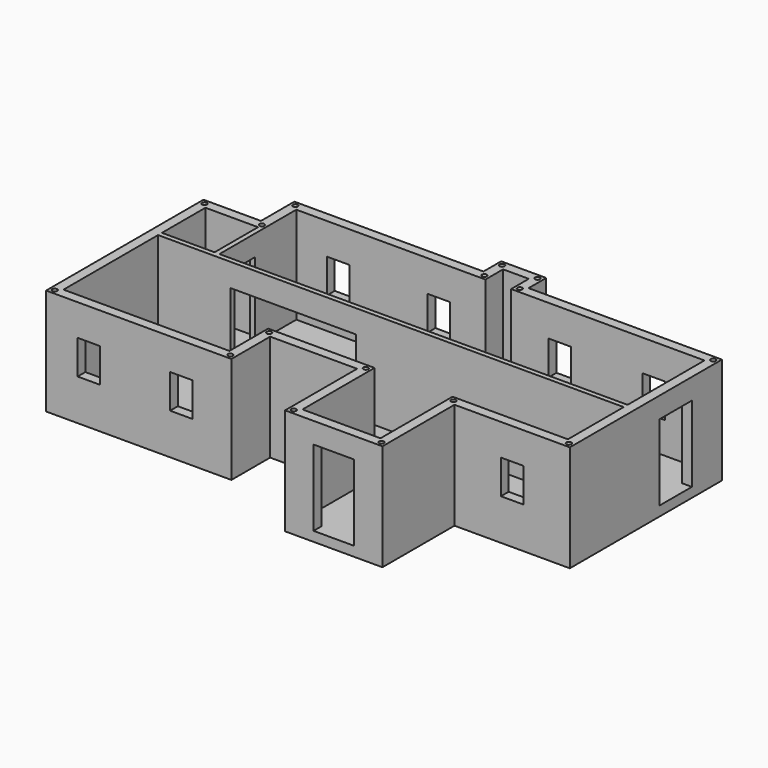
from build123d import *

# Parameters (mm, degrees)
F0_R      = 0.6477
F0_R_2    = 0.6441405576
F0_W      = 1.27
F0_H      = 14.2598937347
F2_DEPTH  = 25.4
F12_DEPTH = 2.54
F4_W      = 5.8928
F4_H      = 8.9408
F3_W      = 5.8928
F3_H      = 8.9408
F13_DEPTH = 25.4
F6_W      = 5.8928
F6_H      = 8.9408
F5_W      = 10.5937230855
F5_H      = 19.9419036508
F7_W      = 5.8928
F7_H      = 8.9408
F14_DEPTH = 12.7
F10_W     = 10.5918
F10_H     = 19.939
F15_DEPTH = 12.7
F9_W      = 10.5918
F9_H      = 19.939
F16_DEPTH = 25.4
F8_W      = 32.9645648599
F8_H      = 19.3392261863
F17_DEPTH = 12.7


# Not quite as in the source:
# - the program builds the solid bodies; features that only make, move or delete a surface that nothing else refers to are left out


with BuildPart() as f2:
    # F0 (on Top) → F2 (new body)
    with BuildSketch(Plane.XY):
        Polygon((-45.4049956864, 2.54), (-47.9449956864, 2.54), (-47.9449956864, 0), (-47.9449956864, -8.4182334522), (-60.4807920754, -8.4182334522), (-63.0207920754, -8.4182334522), (-63.0207920754, -10.9582334522), (-63.0207920754, -57.4975824572), (-63.0207920754, -60.0375824572), (-60.4807920754, -60.0375824572), (-16.9454139954, -60.0375824572), (-14.4054139954, -60.0375824572), (-14.4054139954, -57.4975824572), (-14.4054139954, -47.3375824572), (8.416604454, -47.3375824572), (8.416604454, -68.4223124651), (8.416604454, -70.9623124651), (10.956604454, -70.9623124651), (31.4210504293, -70.9623124651), (33.9610504293, -70.9623124651), (33.9610504293, -68.4223124651), (33.9610504293, -47.3375824572), (61.6818144917, -47.3375824572), (64.2218144917, -47.3375824572), (64.2218144917, -44.7975824572), (64.2218144917, 0), (64.2218144917, 2.54), (61.6818144917, 2.54), (13.496604454, 2.54), (13.496604454, 5.7937128431), (13.496604454, 8.3337128431), (10.956604454, 8.3337128431), (4.2076310147, 8.3337128431), (1.6676310147, 8.3337128431), (1.6676310147, 5.7937128431), (1.6676310147, 2.54), align=None)
        with Locations((-61.7507920754, -58.7675824572)):
            Circle(F0_R, mode=Mode.SUBTRACT)
        with Locations((-15.6754139954, -58.7675824572)):
            Circle(F0_R, mode=Mode.SUBTRACT)
        with Locations((-15.6754139954, -46.0675824572)):
            Circle(F0_R, mode=Mode.SUBTRACT)
        with Locations((9.686604454, -69.6923124651)):
            Circle(F0_R, mode=Mode.SUBTRACT)
        with Locations((32.6910504293, -69.6923124651)):
            Circle(F0_R, mode=Mode.SUBTRACT)
        with Locations((9.686604454, -46.0675824572)):
            Circle(F0_R, mode=Mode.SUBTRACT)
        with Locations((32.6910504293, -46.0675824572)):
            Circle(F0_R, mode=Mode.SUBTRACT)
        with Locations((62.9518144917, -46.0675824572)):
            Circle(F0_R, mode=Mode.SUBTRACT)
        with Locations((-61.7507920754, -9.6882334522)):
            Circle(F0_R, mode=Mode.SUBTRACT)
        with Locations((-46.6749956864, -9.6882334522)):
            Circle(F0_R, mode=Mode.SUBTRACT)
        with Locations((-46.6749956864, 1.27)):
            Circle(F0_R_2, mode=Mode.SUBTRACT)
        Polygon((10.956604454, -68.4223124651), (10.956604454, -47.3375824572), (10.956604454, -44.7975824572), (8.416604454, -44.7975824572), (-14.4054139954, -44.7975824572), (-16.9454139954, -44.7975824572), (-16.9454139954, -47.3375824572), (-16.9454139954, -57.4975824572), (-60.4807920754, -57.4975824572), (-60.4807920754, -26.4881271869), (-60.4807920754, -25.2181271869), (-60.4807920754, -10.9582334522), (-47.9449956864, -10.9582334522), (-46.6749956864, -10.9582334522), (-45.4049956864, -10.9582334522), (-45.4049956864, -8.4182334522), (-45.4049956864, 0), (1.6676310147, 0), (4.2076310147, 0), (4.2076310147, 2.54), (4.2076310147, 5.7937128431), (10.956604454, 5.7937128431), (10.956604454, 2.54), (10.956604454, 0), (13.496604454, 0), (61.6818144917, 0), (61.6818144917, -25.2181271869), (61.6818144917, -26.4881271869), (61.6818144917, -44.7975824572), (33.9610504293, -44.7975824572), (31.4210504293, -44.7975824572), (31.4210504293, -47.3375824572), (31.4210504293, -68.4223124651), align=None, mode=Mode.SUBTRACT)
        with Locations((2.9376310147, 1.27)):
            Circle(F0_R, mode=Mode.SUBTRACT)
        with Locations((12.226604454, 1.27)):
            Circle(F0_R, mode=Mode.SUBTRACT)
        with Locations((2.9376310147, 7.0637128431)):
            Circle(F0_R, mode=Mode.SUBTRACT)
        with Locations((12.226604454, 7.0637128431)):
            Circle(F0_R, mode=Mode.SUBTRACT)
        with Locations((62.9518144917, 1.27)):
            Circle(F0_R, mode=Mode.SUBTRACT)
        Polygon((-60.4807920754, -26.4881271869), (61.6818144917, -26.4881271869), (61.6818144917, -25.2181271869), (-45.4049956864, -25.2181271869), (-46.6749956864, -25.2181271869), (-60.4807920754, -25.2181271869), align=None)
        with Locations((-46.0399956864, -18.0881803195)):
            Rectangle(F0_W, F0_H)
    extrude(amount=F2_DEPTH)

    # F11 (on face) → F12 (join)
    with BuildSketch(Plane(origin=(0, 0, 0), x_dir=(1, 0, 0), z_dir=(0, 0, -1))):
        Polygon((13.496604454, -8.3337128431), (13.496604454, -2.54), (64.2218144917, -2.54), (64.2218144917, 47.3375824572), (33.9610504293, 47.3375824572), (33.9610504293, 70.9623124651), (8.416604454, 70.9623124651), (8.416604454, 47.3375824572), (-14.4054139954, 47.3375824572), (-14.4054139954, 60.0375824572), (-63.0207920754, 60.0375824572), (-63.0207920754, 8.4182334522), (-47.9449956864, 8.4182334522), (-47.9449956864, -2.54), (1.6676310147, -2.54), (1.6676310147, -8.3337128431), align=None)
    extrude(amount=F12_DEPTH)

    # F4 (on face) + F3 (on face) → F13 (cut)
    with BuildSketch(Plane.XZ):
        with Locations((48.364430666, 12.7)):
            Rectangle(F4_W, F4_H)
        with Locations((23.7640291452, 12.7)):
            Rectangle(F4_W, F4_H)
    with BuildSketch(Plane.XZ):
        with Locations((-7.994512096, 12.7)):
            Rectangle(F3_W, F3_H)
        with Locations((-34.4051830471, 12.7)):
            Rectangle(F3_W, F3_H)
    extrude(amount=-F13_DEPTH, mode=Mode.SUBTRACT)

    # F6 (on face) + F5 (on face) + F7 (on face) → F14 (cut)
    with BuildSketch(Plane.XZ.offset(47.3375824572)):
        with Locations((49.0914324605, 12.7)):
            Rectangle(F6_W, F6_H)
    with BuildSketch(Plane.XZ.offset(70.9623124651)):
        with Locations((21.1888274417, 9.9709518254)):
            Rectangle(F5_W, F5_H)
    with BuildSketch(Plane.XZ.offset(60.0375824572)):
        with Locations((-27.5427140296, 12.7)):
            Rectangle(F7_W, F7_H)
        with Locations((-51.7941080034, 12.7)):
            Rectangle(F7_W, F7_H)
    extrude(amount=-F14_DEPTH, mode=Mode.SUBTRACT)

    # F10 (on face) → F15 (cut)
    with BuildSketch(Plane.YZ.offset(-45.4049956864)):
        with Locations((-18.8149667105, 9.9695)):
            Rectangle(F10_W, F10_H)
    extrude(amount=-F15_DEPTH, mode=Mode.SUBTRACT)

    # F9 (on face) → F16 (cut)
    with BuildSketch(Plane(origin=(61.6818144917, 0, 0), x_dir=(0, -1, 0), z_dir=(-1, 0, 0))):
        with Locations((12.6090635934, 9.9695)):
            Rectangle(F9_W, F9_H)
    extrude(amount=-F16_DEPTH, mode=Mode.SUBTRACT)

    # F8 (on face) → F17 (cut)
    with BuildSketch(Plane.XZ.offset(26.4881271869)):
        with Locations((-24.977594614, 9.6696130931)):
            Rectangle(F8_W, F8_H)
    extrude(amount=-F17_DEPTH, mode=Mode.SUBTRACT)


solid = f2.part
